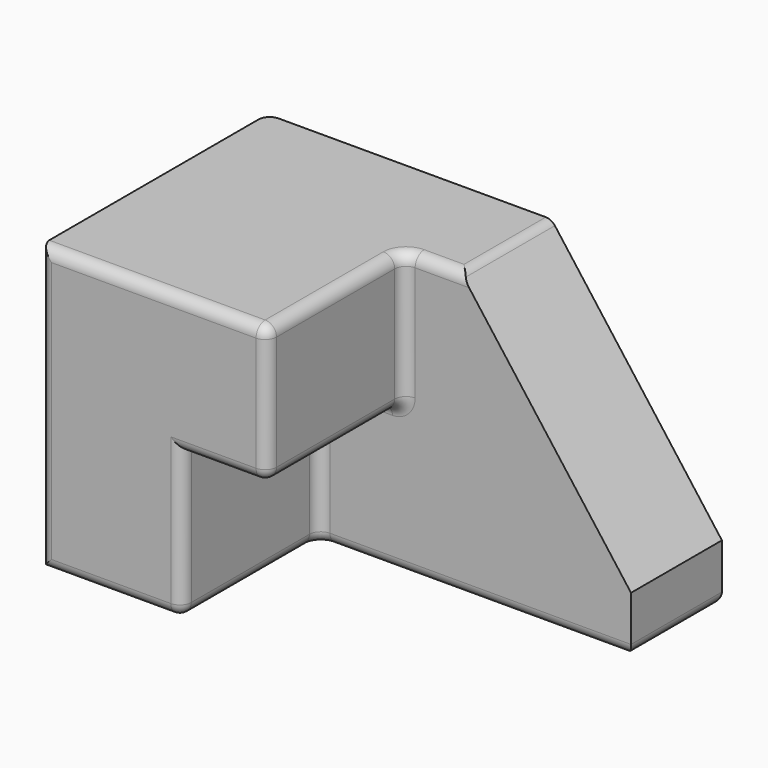
from build123d import *

# Parameters (mm, degrees)
F0_W     = 203.2
F0_H     = 127
F1_DEPTH = 127
F3_DEPTH = 76.2
F4_SIZE2 = 101.6
F4_SIZE  = 76.2
F5_R     = 5.08


with BuildPart() as f1:
    # F0 (on Front) → F1 (new body)
    with BuildSketch(Plane.XZ):
        with Locations((8.8248885557, -5.8830874041)):
            Rectangle(F0_W, F0_H)
    extrude(amount=F1_DEPTH)

    # F2 (on face) → F3 (cut)
    with BuildSketch(Plane.XZ.offset(127)):
        Polygon((110.4248885557, 57.6169125959), (8.8248885557, 57.6169125959), (8.8248885557, -3.765176516), (-29.2751114443, -3.765176516), (-29.2751114443, -69.3830874041), (110.4248885557, -69.3830874041), align=None)
    extrude(amount=-F3_DEPTH, mode=Mode.SUBTRACT)

    # F4
    f4_edges = [f1.edges().sort_by_distance(p)[0] for p in [
        (110.424889, -25.4, 57.616913),
    ]]
    f4_side = f1.faces().sort_by_distance((-12.94654, -52.614286, 57.616913))[0]
    chamfer(f4_edges, length=F4_SIZE, length2=F4_SIZE2, reference=f4_side)

    # F5
    f5_edges = [f1.edges().sort_by_distance(p)[0] for p in [
        (-41.975111, -127, 57.616913),
        (8.824889, -88.9, 57.616913),
        (21.524889, -50.8, 57.616913),
        (34.224889, -25.4, 57.616913),
        (8.824889, -50.8, 26.925868),
        (8.824889, -127, 26.925868),
        (-10.225111, -127, -3.765177),
        (8.824889, -88.9, -3.765177),
        (-29.275111, -127, -36.574132),
        (-29.275111, -50.8, -36.574132),
        (-61.025111, -127, -69.383087),
        (-29.275111, -88.9, -69.383087),
        (40.574889, -50.8, -69.383087),
        (110.424889, -25.4, -69.383087),
        (-92.775111, -127, -5.883087),
        (8.824889, 0, -69.383087),
        (-92.775111, 0, -5.883087),
        (-10.225111, -50.8, -3.765177),
    ]]
    fillet(f5_edges, radius=F5_R)


solid = f1.part
